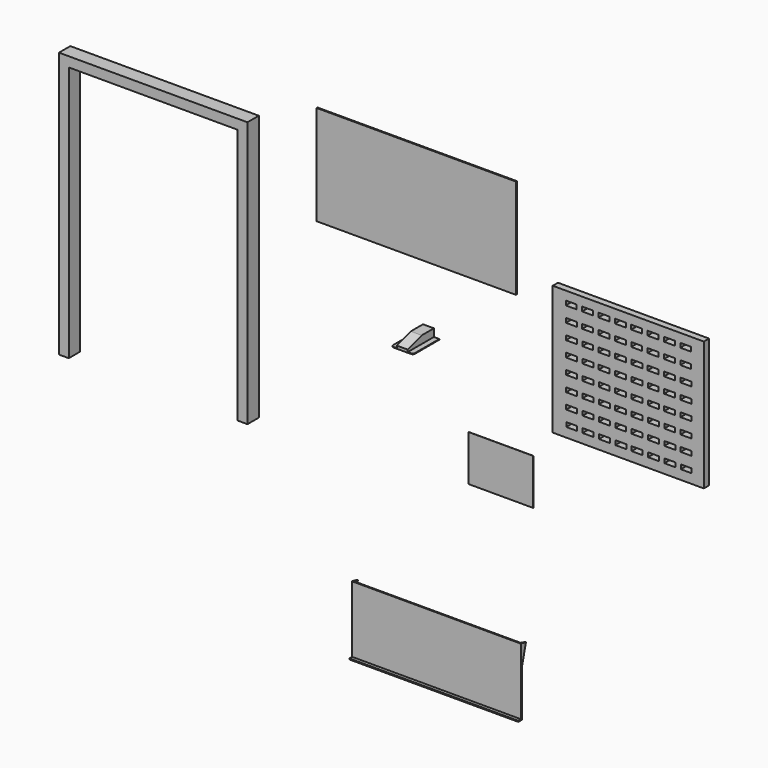
from build123d import *

# Parameters (mm, degrees)
F0_W      = 100
F0_H      = 150
F1_DEPTH  = 3
F2_R      = 10
F3_W      = 50
F3_H      = 150
F4_DEPTH  = 35
F6_DEPTH  = 75.001
F8_DEPTH  = 65
F9_W      = 693
F9_H      = 593
F9_W_2    = 50
F9_H_2    = 20
F10_DEPTH = 30
F9_W_3    = 774.4
F9_H_3    = 304.8
F11_DEPTH = 4.76
F12_W     = 774.4
F12_H     = 4.76
F13_DEPTH = 20
F15_DEPTH = 4
F17_DEPTH = 4.76
F18_W     = 914.4
F18_H     = 457.2
F19_DEPTH = 5
F20_W     = 297
F20_H     = 210
F21_DEPTH = 1


# Not quite as in the source:
# - a feature names something its author has since deleted; it is built from what else it names


with BuildPart() as f1:
    # F0 (on Top) → F1 (new body)
    with BuildSketch(Plane.XY):
        Rectangle(F0_W, F0_H)
    extrude(amount=F1_DEPTH)

    # F2
    f2_edges = [f1.edges().sort_by_distance(p)[0] for p in [
        (-50, -75, 1.5),
        (50, -75, 1.5),
    ]]
    fillet(f2_edges, radius=F2_R)

    # F3 (on face) → F4 (join)
    with BuildSketch(Plane.XY.offset(3)):
        Rectangle(F3_W, F3_H)
    extrude(amount=F4_DEPTH)

    # F5 (on face) → F6 (cut, through all)
    with BuildSketch(Plane.YZ.offset(25)):
        Polygon((-75, 13), (5, 38), (-75, 38), align=None)
    extrude(amount=-F6_DEPTH, mode=Mode.SUBTRACT)


with BuildPart() as f8:
    # F7 (on Front) → F8 (new body)
    with BuildSketch(Plane.XZ):
        Polygon((-1582.4594926834, 685.0416660309), (-1582.4594926834, -533.9583339691), (-1537.4594926834, -533.9583339691), (-1537.4594926834, 640.0416660309), (-763.0594926834, 640.0416660309), (-763.0594926834, -533.9583339691), (-718.0594926834, -533.9583339691), (-718.0594926834, 685.0416660309), align=None)
    extrude(amount=F8_DEPTH)


with BuildPart() as f10:
    # F9 (on Front) → F10 (new body)
    with BuildSketch(Plane.XZ):
        with Locations((1000.2106370564, 160.5004700422)):
            Rectangle(F9_W, F9_H)
        with Locations((741.0349838533, -82.9940170818)):
            Rectangle(F9_W_2, F9_H_2, mode=Mode.SUBTRACT)
        with Locations((816.0349838533, -82.9940170818)):
            Rectangle(F9_W_2, F9_H_2, mode=Mode.SUBTRACT)
        with Locations((740.7029343109, -12.9948046355)):
            Rectangle(F9_W_2, F9_H_2, mode=Mode.SUBTRACT)
        with Locations((815.7029343109, -12.9948046355)):
            Rectangle(F9_W_2, F9_H_2, mode=Mode.SUBTRACT)
        with Locations((891.0349838533, -82.9940170818)):
            Rectangle(F9_W_2, F9_H_2, mode=Mode.SUBTRACT)
        with Locations((890.7029343109, -12.9948046355)):
            Rectangle(F9_W_2, F9_H_2, mode=Mode.SUBTRACT)
        with Locations((966.0349838533, -82.9940170818)):
            Rectangle(F9_W_2, F9_H_2, mode=Mode.SUBTRACT)
        with Locations((965.7029343109, -12.9948046355)):
            Rectangle(F9_W_2, F9_H_2, mode=Mode.SUBTRACT)
        with Locations((1041.0349838533, -82.9940170818)):
            Rectangle(F9_W_2, F9_H_2, mode=Mode.SUBTRACT)
        with Locations((1116.0349838533, -82.9940170818)):
            Rectangle(F9_W_2, F9_H_2, mode=Mode.SUBTRACT)
        with Locations((1040.7029343109, -12.9948046355)):
            Rectangle(F9_W_2, F9_H_2, mode=Mode.SUBTRACT)
        with Locations((1115.7029343109, -12.9948046355)):
            Rectangle(F9_W_2, F9_H_2, mode=Mode.SUBTRACT)
        with Locations((1191.0349838533, -82.9940170818)):
            Rectangle(F9_W_2, F9_H_2, mode=Mode.SUBTRACT)
        with Locations((1190.7029343109, -12.9948046355)):
            Rectangle(F9_W_2, F9_H_2, mode=Mode.SUBTRACT)
        with Locations((1266.0349838533, -82.9940170818)):
            Rectangle(F9_W_2, F9_H_2, mode=Mode.SUBTRACT)
        with Locations((1265.7029343109, -12.9948046355)):
            Rectangle(F9_W_2, F9_H_2, mode=Mode.SUBTRACT)
        with Locations((740.3708847685, 57.0044078108)):
            Rectangle(F9_W_2, F9_H_2, mode=Mode.SUBTRACT)
        with Locations((815.3708847685, 57.0044078108)):
            Rectangle(F9_W_2, F9_H_2, mode=Mode.SUBTRACT)
        with Locations((890.3708847685, 57.0044078108)):
            Rectangle(F9_W_2, F9_H_2, mode=Mode.SUBTRACT)
        with Locations((740.0388352261, 127.0036202571)):
            Rectangle(F9_W_2, F9_H_2, mode=Mode.SUBTRACT)
        with Locations((815.038835226, 127.0036202571)):
            Rectangle(F9_W_2, F9_H_2, mode=Mode.SUBTRACT)
        with Locations((739.7067856836, 197.0028327033)):
            Rectangle(F9_W_2, F9_H_2, mode=Mode.SUBTRACT)
        with Locations((814.7067856836, 197.0028327033)):
            Rectangle(F9_W_2, F9_H_2, mode=Mode.SUBTRACT)
        with Locations((890.038835226, 127.0036202571)):
            Rectangle(F9_W_2, F9_H_2, mode=Mode.SUBTRACT)
        with Locations((889.7067856836, 197.0028327033)):
            Rectangle(F9_W_2, F9_H_2, mode=Mode.SUBTRACT)
        with Locations((739.3747361412, 267.0020451496)):
            Rectangle(F9_W_2, F9_H_2, mode=Mode.SUBTRACT)
        with Locations((814.3747361412, 267.0020451496)):
            Rectangle(F9_W_2, F9_H_2, mode=Mode.SUBTRACT)
        with Locations((739.0426865988, 337.0012575959)):
            Rectangle(F9_W_2, F9_H_2, mode=Mode.SUBTRACT)
        with Locations((814.0426865988, 337.0012575959)):
            Rectangle(F9_W_2, F9_H_2, mode=Mode.SUBTRACT)
        with Locations((889.3747361412, 267.0020451496)):
            Rectangle(F9_W_2, F9_H_2, mode=Mode.SUBTRACT)
        with Locations((889.0426865988, 337.0012575959)):
            Rectangle(F9_W_2, F9_H_2, mode=Mode.SUBTRACT)
        with Locations((738.7106370564, 407.0004700422)):
            Rectangle(F9_W_2, F9_H_2, mode=Mode.SUBTRACT)
        with Locations((813.7106370564, 407.0004700422)):
            Rectangle(F9_W_2, F9_H_2, mode=Mode.SUBTRACT)
        with Locations((888.7106370564, 407.0004700422)):
            Rectangle(F9_W_2, F9_H_2, mode=Mode.SUBTRACT)
        with Locations((965.3708847685, 57.0044078108)):
            Rectangle(F9_W_2, F9_H_2, mode=Mode.SUBTRACT)
        with Locations((1040.3708847685, 57.0044078108)):
            Rectangle(F9_W_2, F9_H_2, mode=Mode.SUBTRACT)
        with Locations((1115.3708847685, 57.0044078108)):
            Rectangle(F9_W_2, F9_H_2, mode=Mode.SUBTRACT)
        with Locations((965.038835226, 127.0036202571)):
            Rectangle(F9_W_2, F9_H_2, mode=Mode.SUBTRACT)
        with Locations((1040.038835226, 127.0036202571)):
            Rectangle(F9_W_2, F9_H_2, mode=Mode.SUBTRACT)
        with Locations((964.7067856836, 197.0028327033)):
            Rectangle(F9_W_2, F9_H_2, mode=Mode.SUBTRACT)
        with Locations((1039.7067856836, 197.0028327033)):
            Rectangle(F9_W_2, F9_H_2, mode=Mode.SUBTRACT)
        with Locations((1115.038835226, 127.0036202571)):
            Rectangle(F9_W_2, F9_H_2, mode=Mode.SUBTRACT)
        with Locations((1114.7067856836, 197.0028327033)):
            Rectangle(F9_W_2, F9_H_2, mode=Mode.SUBTRACT)
        with Locations((1190.3708847685, 57.0044078108)):
            Rectangle(F9_W_2, F9_H_2, mode=Mode.SUBTRACT)
        with Locations((1265.3708847685, 57.0044078108)):
            Rectangle(F9_W_2, F9_H_2, mode=Mode.SUBTRACT)
        with Locations((1190.038835226, 127.0036202571)):
            Rectangle(F9_W_2, F9_H_2, mode=Mode.SUBTRACT)
        with Locations((1189.7067856836, 197.0028327033)):
            Rectangle(F9_W_2, F9_H_2, mode=Mode.SUBTRACT)
        with Locations((1265.038835226, 127.0036202571)):
            Rectangle(F9_W_2, F9_H_2, mode=Mode.SUBTRACT)
        with Locations((1264.7067856836, 197.0028327033)):
            Rectangle(F9_W_2, F9_H_2, mode=Mode.SUBTRACT)
        with Locations((964.3747361412, 267.0020451496)):
            Rectangle(F9_W_2, F9_H_2, mode=Mode.SUBTRACT)
        with Locations((1039.3747361412, 267.0020451496)):
            Rectangle(F9_W_2, F9_H_2, mode=Mode.SUBTRACT)
        with Locations((964.0426865988, 337.0012575959)):
            Rectangle(F9_W_2, F9_H_2, mode=Mode.SUBTRACT)
        with Locations((1039.0426865988, 337.0012575959)):
            Rectangle(F9_W_2, F9_H_2, mode=Mode.SUBTRACT)
        with Locations((1114.3747361412, 267.0020451496)):
            Rectangle(F9_W_2, F9_H_2, mode=Mode.SUBTRACT)
        with Locations((1114.0426865988, 337.0012575959)):
            Rectangle(F9_W_2, F9_H_2, mode=Mode.SUBTRACT)
        with Locations((963.7106370564, 407.0004700422)):
            Rectangle(F9_W_2, F9_H_2, mode=Mode.SUBTRACT)
        with Locations((1038.7106370564, 407.0004700422)):
            Rectangle(F9_W_2, F9_H_2, mode=Mode.SUBTRACT)
        with Locations((1113.7106370564, 407.0004700422)):
            Rectangle(F9_W_2, F9_H_2, mode=Mode.SUBTRACT)
        with Locations((1189.3747361412, 267.0020451496)):
            Rectangle(F9_W_2, F9_H_2, mode=Mode.SUBTRACT)
        with Locations((1189.0426865988, 337.0012575959)):
            Rectangle(F9_W_2, F9_H_2, mode=Mode.SUBTRACT)
        with Locations((1264.3747361412, 267.0020451496)):
            Rectangle(F9_W_2, F9_H_2, mode=Mode.SUBTRACT)
        with Locations((1264.0426865988, 337.0012575959)):
            Rectangle(F9_W_2, F9_H_2, mode=Mode.SUBTRACT)
        with Locations((1188.7106370564, 407.0004700422)):
            Rectangle(F9_W_2, F9_H_2, mode=Mode.SUBTRACT)
        with Locations((1263.7106370564, 407.0004700422)):
            Rectangle(F9_W_2, F9_H_2, mode=Mode.SUBTRACT)
    extrude(amount=F10_DEPTH)


with BuildPart() as f11:
    # F9 (on Front) → F11 (new body)
    with BuildSketch(Plane.XZ):
        with Locations((100.6992778301, -1204.7096658707)):
            Rectangle(F9_W_3, F9_H_3)
    extrude(amount=F11_DEPTH)

    # F12 (on face) → F13 (join)
    with BuildSketch(Plane.XZ):
        with Locations((100.6992778301, -1359.4896658707)):
            Rectangle(F12_W, F12_H)
    extrude(amount=F13_DEPTH)

    # F14 (on face) → F15 (join)
    with BuildSketch(Plane(origin=(-286.5007221699, 0, 0), x_dir=(0, -1, 0), z_dir=(-1, 0, 0))):
        Polygon((0, -1153.309801547), (0, -1052.3096658707), (-23.7083457688, -1058.2208203719), align=None)
    extrude(amount=-F15_DEPTH)

    # F16 (on face) → F17 (join)
    with BuildSketch(Plane.YZ.offset(487.8992778301)):
        Polygon((23.7083457688, -1058.2208203719), (0, -1052.3096658707), (0, -1153.309801547), align=None)
    extrude(amount=-F17_DEPTH)


with BuildPart() as f19:
    # F18 (on Front) → F19 (new body)
    with BuildSketch(Plane.XZ):
        with Locations((7.7835917473, 577.2774274308)):
            Rectangle(F18_W, F18_H)
    extrude(amount=F19_DEPTH)


with BuildPart() as f21:
    # F20 (on Front) → F21 (new body)
    with BuildSketch(Plane.XZ):
        with Locations((392.1522349119, -383.521551521)):
            Rectangle(F20_W, F20_H)
    extrude(amount=F21_DEPTH)


solid = Compound([f1.part, f8.part, f10.part, f11.part, f19.part, f21.part])
